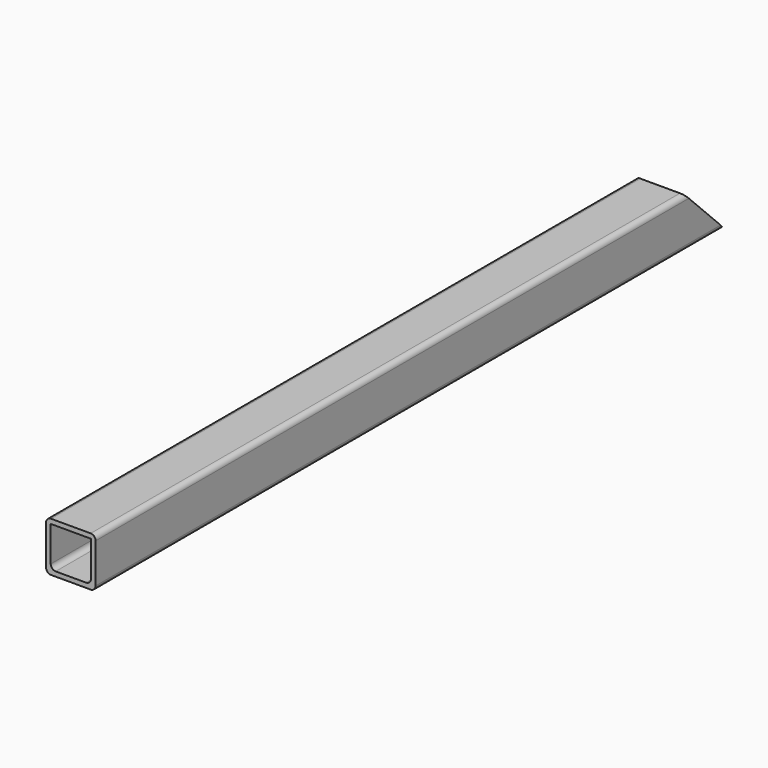
from build123d import *

# Parameters (mm, degrees)
F0_W     = 50.8
F0_H     = 50.8
F0_W_2   = 41.275
F0_H_2   = 41.275
F1_DEPTH = 403.225
F3_DEPTH = 50.8
F4_R     = 5.08


with BuildPart() as f1:
    # F0 (on Front) → F1 (new body, symmetric)
    with BuildSketch(Plane.XZ):
        Rectangle(F0_W, F0_H)
        Rectangle(F0_W_2, F0_H_2, mode=Mode.SUBTRACT)
    extrude(amount=F1_DEPTH, both=True)

    # F2 (on face) → F3 (cut)
    with BuildSketch(Plane(origin=(-25.4, 0, 0), x_dir=(0, -1, 0), z_dir=(-1, 0, 0))):
        Polygon((-352.425, 25.4), (-403.225, 25.4), (-403.225, -25.4), align=None)
    extrude(amount=-F3_DEPTH, mode=Mode.SUBTRACT)

    # F4
    f4_edges = [f1.edges().sort_by_distance(p)[0] for p in [
        (-25.4, -25.4, 25.4),
        (25.4, -25.4, 25.4),
        (20.6375, -2.38125, -20.6375),
        (-20.6375, -2.38125, -20.6375),
        (-25.4, 0, -25.4),
        (25.4, 0, -25.4),
    ]]
    fillet(f4_edges, radius=F4_R)


solid = f1.part
